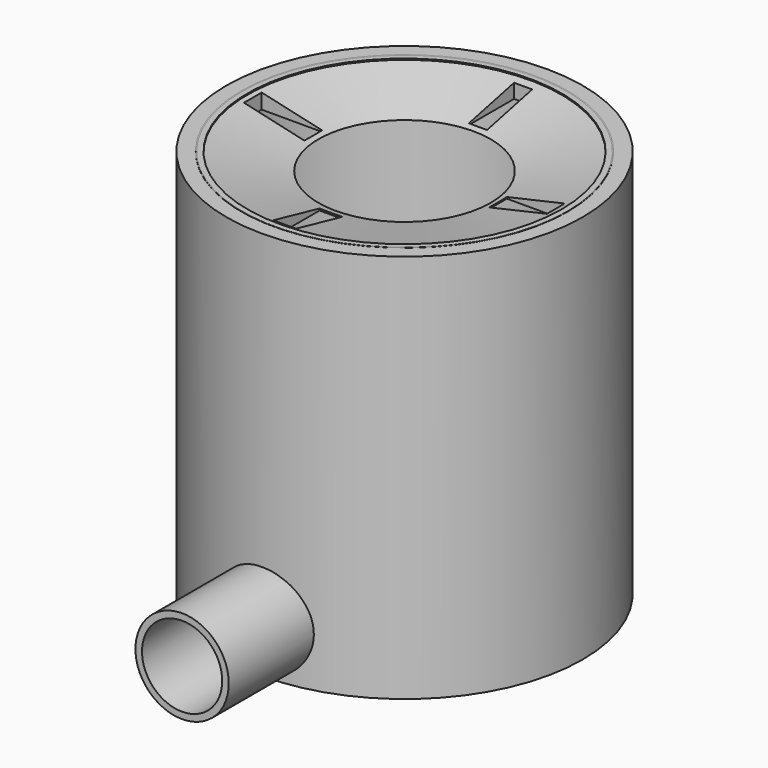
from build123d import *

# Parameters (mm, degrees)
F0_R      = 82.55
F1_DEPTH  = 196.85
F2_R      = 79.375
F3_DEPTH  = 190.5
F9_W      = 9.1596553102
F9_H      = 28.4967124462
F9_W_2    = 29.1752070189
F9_H_2    = 11.1951339059
F9_W_3    = 30.5321961641
F9_H_3    = 11.1951371655
F9_W_4    = 11.5343825892
F9_H_4    = 29.1751995683
F10_DEPTH = 50.8
F11_R     = 23.5856126994
F12_DEPTH = 140.54548
F13_R     = 20.2662897719
F14_DEPTH = 100.21757
F15_R     = 90.0641643282
F15_R_2   = 82.55
F16_DEPTH = 196.85


# Not quite as in the source:
# - the program builds the solid bodies; features that only make, move or delete a surface that nothing else refers to are left out


with BuildPart() as f1:
    # F0 (on Top) → F1 (new body)
    with BuildSketch(Plane.XY):
        Circle(F0_R)
    extrude(amount=F1_DEPTH)

    # F2 (on face) → F3 (cut)
    with BuildSketch(Plane.XY.offset(196.85)):
        Circle(F2_R)
    extrude(amount=-F3_DEPTH, mode=Mode.SUBTRACT)

    # F7 (on Front) → F8 (revolve)
    with BuildSketch(Plane.XZ):
        Polygon((82.5372104228, 188.0925446749), (82.5032889843, 196.9533860683), (43.5591638088, 188.0925446749), align=None)
    revolve(axis=Axis((0, 0, 196.85), (0, 0, 1)))

    # F9 (on offset) → F10 (cut)
    with BuildSketch(Plane.XY.offset(196.85)):
        with Locations((-0.1696236432, 60.8947575092)):
            Rectangle(F9_W, F9_H)
        with Locations((60.8947575092, 1.187362941)):
            Rectangle(F9_W_2, F9_H_2)
        with Locations((-61.5732520819, 0.1696236432)):
            Rectangle(F9_W_3, F9_H_3)
        with Locations((0.6784931757, -61.9124956429)):
            Rectangle(F9_W_4, F9_H_4)
    extrude(amount=-F10_DEPTH, mode=Mode.SUBTRACT)

    # F11 (on Front) → F12 (join)
    with BuildSketch(Plane.XZ):
        with Locations((0, 24.8852539808)):
            Circle(F11_R)
    extrude(amount=F12_DEPTH)

    # F13 (on face) → F14 (cut)
    with BuildSketch(Plane.XZ.offset(140.54548)):
        with Locations((0, 24.8852539808)):
            Circle(F13_R)
    extrude(amount=-F14_DEPTH, mode=Mode.SUBTRACT)


with BuildPart() as f16:
    # F15 (on Top) → F16 (new body)
    with BuildSketch(Plane.XY):
        Circle(F15_R)
        Circle(F15_R_2, mode=Mode.SUBTRACT)
    extrude(amount=F16_DEPTH)


solid = Compound([f1.part, f16.part])
